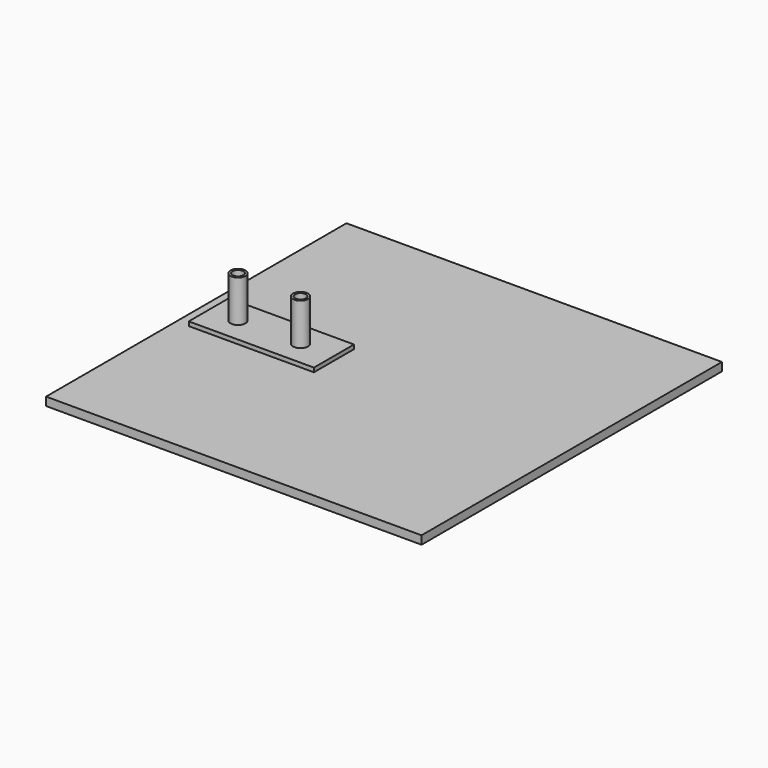
from build123d import *

# Parameters (mm, degrees)
F0_R     = 1.8
F0_R_2   = 1.3
F1_DEPTH = 13
F0_W     = 30
F0_H     = 12
F2_DEPTH = 3
F0_W_2   = 90
F0_H_2   = 90
F3_DEPTH = 2


with BuildPart() as f1:
    # F0 (on Top) → F1 (new body)
    with BuildSketch(Plane.XY):
        with Locations((-35, 0)):
            Circle(F0_R)
        with Locations((-35, 0)):
            Circle(F0_R_2, mode=Mode.SUBTRACT)
    extrude(amount=F1_DEPTH)



with BuildPart() as f1b:
    # F0 (on Top) → F1, piece 2 (new body)
    with BuildSketch(Plane.XY):
        with Locations((-20, 0)):
            Circle(F0_R)
        with Locations((-20, 0)):
            Circle(F0_R_2, mode=Mode.SUBTRACT)
    extrude(amount=F1_DEPTH)


with BuildPart() as f1_1:
    add(f1.part)

    add(f1b.part)  # F2 merges F1b
    # F0 (on Top) → F2 (join)
    with BuildSketch(Plane.XY):
        with Locations((-27, 0)):
            Rectangle(F0_W, F0_H)
        with Locations((-35, 0)):
            Circle(F0_R, mode=Mode.SUBTRACT)
        with Locations((-20, 0)):
            Circle(F0_R, mode=Mode.SUBTRACT)
        with Locations((-20, 0)):
            Circle(F0_R_2)
        with Locations((-35, 0)):
            Circle(F0_R_2)
    extrude(amount=F2_DEPTH)

    # F0 (on Top) → F3 (join)
    with BuildSketch(Plane.XY):
        Rectangle(F0_W_2, F0_H_2)
        with Locations((-27, 0)):
            Rectangle(F0_W, F0_H, mode=Mode.SUBTRACT)
    extrude(amount=F3_DEPTH)


solid = f1_1.part
